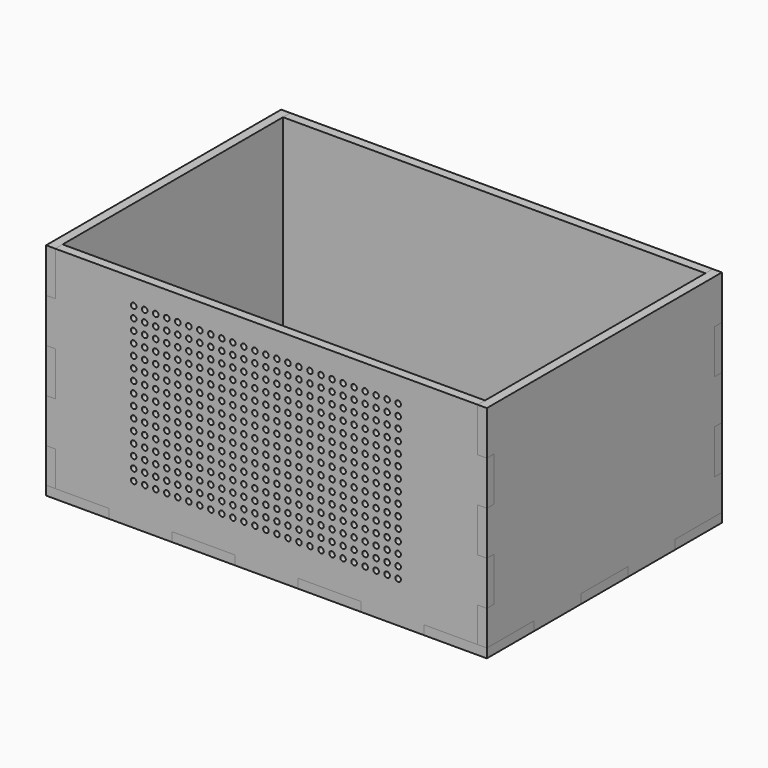
from build123d import *

# Parameters (mm, degrees)
F0_W      = 18.5964285714
F0_H      = 3.175
F0_W_2    = 3.175
F0_H_2    = 17.145
F0_H_3    = 20.32
F0_W_3    = 21.7714285714
F1_DEPTH  = 3.175
F2_W      = 3.175
F2_H      = 15.24
F2_H_2    = 12.065
F2_H_3    = 3.175
F3_DEPTH  = 3.175
F7_DEPTH  = 3.175
F10_R     = 0.9525
F11_DEPTH = 25.4


with BuildPart() as f1:
    # F0 (on Top) → F1 (new body)
    with BuildSketch(Plane.XY):
        Polygon((73.025, 30.48), (73.025, 47.625), (54.4285714286, 47.625), (32.6571428571, 47.625), (10.8857142857, 47.625), (-10.8857142857, 47.625), (-32.6571428571, 47.625), (-54.4285714286, 47.625), (-73.025, 47.625), (-73.025, 30.48), (-73.025, 10.16), (-73.025, -10.16), (-73.025, -30.48), (-73.025, -47.625), (-54.4285714286, -47.625), (-32.6571428571, -47.625), (-10.8857142857, -47.625), (10.8857142857, -47.625), (32.6571428571, -47.625), (54.4285714286, -47.625), (73.025, -47.625), (73.025, -30.48), (73.025, -10.16), (73.025, 10.16), align=None)
        with Locations((-63.7267857143, 49.2125)):
            Rectangle(F0_W, F0_H)
        with Locations((-74.6125, 49.2125)):
            Rectangle(F0_W_2, F0_H)
        with Locations((-74.6125, 39.0525)):
            Rectangle(F0_W_2, F0_H_2)
        with Locations((-74.6125, 0)):
            Rectangle(F0_W_2, F0_H_3)
        with Locations((-74.6125, -39.0525)):
            Rectangle(F0_W_2, F0_H_2)
        with Locations((-74.6125, -49.2125)):
            Rectangle(F0_W_2, F0_H)
        with Locations((-63.7267857143, -49.2125)):
            Rectangle(F0_W, F0_H)
        with Locations((-21.7714285714, -49.2125)):
            Rectangle(F0_W_3, F0_H)
        with Locations((21.7714285714, -49.2125)):
            Rectangle(F0_W_3, F0_H)
        with Locations((63.7267857143, -49.2125)):
            Rectangle(F0_W, F0_H)
        with Locations((74.6125, -49.2125)):
            Rectangle(F0_W_2, F0_H)
        with Locations((74.6125, -39.0525)):
            Rectangle(F0_W_2, F0_H_2)
        with Locations((74.6125, 0)):
            Rectangle(F0_W_2, F0_H_3)
        with Locations((74.6125, 39.0525)):
            Rectangle(F0_W_2, F0_H_2)
        with Locations((74.6125, 49.2125)):
            Rectangle(F0_W_2, F0_H)
        with Locations((63.7267857143, 49.2125)):
            Rectangle(F0_W, F0_H)
        with Locations((21.7714285714, 49.2125)):
            Rectangle(F0_W_3, F0_H)
        with Locations((-21.7714285714, 49.2125)):
            Rectangle(F0_W_3, F0_H)
    extrude(amount=F1_DEPTH)


with BuildPart() as f3:
    # F2 (on face) → F3 (new body)
    with BuildSketch(Plane.YZ.offset(76.2)):
        Polygon((-30.48, 3.175), (-30.48, 0), (47.625, 0), (47.625, 15.24), (47.625, 30.48), (47.625, 45.72), (47.625, 60.96), (47.625, 76.2), (-47.625, 76.2), (-47.625, 60.96), (-47.625, 45.72), (-47.625, 30.48), (-47.625, 15.24), (-47.625, 3.175), align=None)
        with Locations((-49.2125, 68.58)):
            Rectangle(F2_W, F2_H)
        with Locations((-49.2125, 38.1)):
            Rectangle(F2_W, F2_H)
        with Locations((-49.2125, 9.2075)):
            Rectangle(F2_W, F2_H_2)
        with Locations((49.2125, 7.62)):
            Rectangle(F2_W, F2_H)
        with Locations((49.2125, 38.1)):
            Rectangle(F2_W, F2_H)
        with Locations((49.2125, 68.58)):
            Rectangle(F2_W, F2_H)
        with Locations((-49.2125, 1.5875)):
            Rectangle(F2_W, F2_H_3)
    extrude(amount=-F3_DEPTH)

    # F4: cut F1
    add(f1.part, mode=Mode.SUBTRACT)


with BuildPart() as f5_1:
    # F5: instance of F3
    add(f3.part.mirror(Plane.YZ))


with BuildPart() as f7:
    # F6 (on face) → F7 (new body)
    with BuildSketch(Plane(origin=(0, 50.8, 0), x_dir=(-1, 0, 0), z_dir=(0, 1, 0))):
        Polygon((-54.4285714286, 3.175), (-54.4285714286, 0), (76.2, 0), (76.2, 76.2), (-76.2, 76.2), (-76.2, 3.175), align=None)
    extrude(amount=-F7_DEPTH)

    # F8: cut F5_1, F1, F3
    add(f5_1.part, mode=Mode.SUBTRACT)
    add(f1.part, mode=Mode.SUBTRACT)
    add(f3.part, mode=Mode.SUBTRACT)


with BuildPart() as f9_1:
    # F9: instance of F7
    add(f7.part.mirror(Plane.XZ))

    # F10 (on face) → F11 (cut)
    with BuildSketch(Plane.XZ.offset(50.8)):
        with Locations((-26.85742952, 18.0873329692)):
            Circle(F10_R)
        with Locations((-30.66742952, 21.8973329692)):
            Circle(F10_R)
        with Locations((-34.47742952, 25.7073329692)):
            Circle(F10_R)
        with Locations((-3.99742952, 56.1873329692)):
            Circle(F10_R)
        with Locations((-7.80742952, 59.9973329692)):
            Circle(F10_R)
        with Locations((-11.61742952, 63.8073329692)):
            Circle(F10_R)
        with Locations((-15.42742952, 67.6173329692)):
            Circle(F10_R)
        with Locations((11.24257048, 40.9473329692)):
            Circle(F10_R)
        with Locations((7.43257048, 44.7573329692)):
            Circle(F10_R)
        with Locations((3.62257048, 48.5673329692)):
            Circle(F10_R)
        with Locations((-0.18742952, 52.3773329692)):
            Circle(F10_R)
        with Locations((26.48257048, 25.7073329692)):
            Circle(F10_R)
        with Locations((22.67257048, 29.5173329692)):
            Circle(F10_R)
        with Locations((15.05257048, 37.1373329692)):
            Circle(F10_R)
        with Locations((45.53257048, 67.6173329692)):
            Circle(F10_R)
        with Locations((34.10257048, 18.0873329692)):
            Circle(F10_R)
        with Locations((30.29257048, 21.8973329692)):
            Circle(F10_R)
        with Locations((-45.90742952, 18.0873329692)):
            Circle(F10_R)
        with Locations((-45.90742952, 59.9973329692)):
            Circle(F10_R)
        with Locations((-45.90742952, 56.1873329692)):
            Circle(F10_R)
        with Locations((-45.90742952, 52.3773329692)):
            Circle(F10_R)
        with Locations((-45.90742952, 40.9473329692)):
            Circle(F10_R)
        with Locations((-45.90742952, 37.1373329692)):
            Circle(F10_R)
        with Locations((-45.90742952, 21.8973329692)):
            Circle(F10_R)
        with Locations((-30.66742952, 18.0873329692)):
            Circle(F10_R)
        with Locations((-34.47742952, 21.8973329692)):
            Circle(F10_R)
        with Locations((-3.99742952, 52.3773329692)):
            Circle(F10_R)
        with Locations((-7.80742952, 56.1873329692)):
            Circle(F10_R)
        with Locations((-11.61742952, 59.9973329692)):
            Circle(F10_R)
        with Locations((-15.42742952, 63.8073329692)):
            Circle(F10_R)
        with Locations((11.24257048, 37.1373329692)):
            Circle(F10_R)
        with Locations((7.43257048, 40.9473329692)):
            Circle(F10_R)
        with Locations((3.62257048, 44.7573329692)):
            Circle(F10_R)
        with Locations((26.48257048, 21.8973329692)):
            Circle(F10_R)
        with Locations((22.67257048, 25.7073329692)):
            Circle(F10_R)
        with Locations((45.53257048, 63.8073329692)):
            Circle(F10_R)
        with Locations((41.72257048, 67.6173329692)):
            Circle(F10_R)
        with Locations((30.29257048, 18.0873329692)):
            Circle(F10_R)
        with Locations((-7.80742952, 52.3773329692)):
            Circle(F10_R)
        with Locations((-11.61742952, 56.1873329692)):
            Circle(F10_R)
        with Locations((-15.42742952, 59.9973329692)):
            Circle(F10_R)
        with Locations((7.43257048, 37.1373329692)):
            Circle(F10_R)
        with Locations((3.62257048, 40.9473329692)):
            Circle(F10_R)
        with Locations((26.48257048, 18.0873329692)):
            Circle(F10_R)
        with Locations((22.67257048, 21.8973329692)):
            Circle(F10_R)
        with Locations((45.53257048, 59.9973329692)):
            Circle(F10_R)
        with Locations((41.72257048, 63.8073329692)):
            Circle(F10_R)
        with Locations((-38.28742952, 21.8973329692)):
            Circle(F10_R)
        with Locations((-30.66742952, 14.2773329692)):
            Circle(F10_R)
        with Locations((-34.47742952, 18.0873329692)):
            Circle(F10_R)
        with Locations((7.43257048, 33.3273329692)):
            Circle(F10_R)
        with Locations((3.62257048, 37.1373329692)):
            Circle(F10_R)
        with Locations((-0.18742952, 40.9473329692)):
            Circle(F10_R)
        with Locations((26.48257048, 14.2773329692)):
            Circle(F10_R)
        with Locations((22.67257048, 18.0873329692)):
            Circle(F10_R)
        with Locations((18.86257048, 21.8973329692)):
            Circle(F10_R)
        with Locations((45.53257048, 56.1873329692)):
            Circle(F10_R)
        with Locations((41.72257048, 59.9973329692)):
            Circle(F10_R)
        with Locations((-38.28742952, 18.0873329692)):
            Circle(F10_R)
        with Locations((-42.09742952, 21.8973329692)):
            Circle(F10_R)
        with Locations((-34.47742952, 14.2773329692)):
            Circle(F10_R)
        with Locations((-11.61742952, 52.3773329692)):
            Circle(F10_R)
        with Locations((-15.42742952, 56.1873329692)):
            Circle(F10_R)
        with Locations((22.67257048, 14.2773329692)):
            Circle(F10_R)
        with Locations((18.86257048, 18.0873329692)):
            Circle(F10_R)
        with Locations((15.05257048, 21.8973329692)):
            Circle(F10_R)
        with Locations((45.53257048, 52.3773329692)):
            Circle(F10_R)
        with Locations((41.72257048, 56.1873329692)):
            Circle(F10_R)
        with Locations((-42.09742952, 18.0873329692)):
            Circle(F10_R)
        with Locations((-19.23742952, 56.1873329692)):
            Circle(F10_R)
        with Locations((-30.66742952, 67.6173329692)):
            Circle(F10_R)
        with Locations((-3.99742952, 40.9473329692)):
            Circle(F10_R)
        with Locations((-11.61742952, 48.5673329692)):
            Circle(F10_R)
        with Locations((-15.42742952, 52.3773329692)):
            Circle(F10_R)
        with Locations((7.43257048, 29.5173329692)):
            Circle(F10_R)
        with Locations((3.62257048, 33.3273329692)):
            Circle(F10_R)
        with Locations((-0.18742952, 37.1373329692)):
            Circle(F10_R)
        with Locations((-30.66742952, 44.7573329692)):
            Circle(F10_R)
        with Locations((-34.47742952, 48.5673329692)):
            Circle(F10_R)
        with Locations((-38.28742952, 52.3773329692)):
            Circle(F10_R)
        with Locations((-42.09742952, 56.1873329692)):
            Circle(F10_R)
        with Locations((-15.42742952, 29.5173329692)):
            Circle(F10_R)
        with Locations((-23.04742952, 37.1373329692)):
            Circle(F10_R)
        with Locations((-26.85742952, 40.9473329692)):
            Circle(F10_R)
        with Locations((-3.99742952, 18.0873329692)):
            Circle(F10_R)
        with Locations((-7.80742952, 21.8973329692)):
            Circle(F10_R)
        with Locations((-11.61742952, 25.7073329692)):
            Circle(F10_R)
        with Locations((18.86257048, 56.1873329692)):
            Circle(F10_R)
        with Locations((7.43257048, 67.6173329692)):
            Circle(F10_R)
        with Locations((34.10257048, 40.9473329692)):
            Circle(F10_R)
        with Locations((26.48257048, 48.5673329692)):
            Circle(F10_R)
        with Locations((22.67257048, 52.3773329692)):
            Circle(F10_R)
        with Locations((45.53257048, 29.5173329692)):
            Circle(F10_R)
        with Locations((41.72257048, 33.3273329692)):
            Circle(F10_R)
        with Locations((37.91257048, 37.1373329692)):
            Circle(F10_R)
        with Locations((-30.66742952, 40.9473329692)):
            Circle(F10_R)
        with Locations((-34.47742952, 44.7573329692)):
            Circle(F10_R)
        with Locations((-42.09742952, 52.3773329692)):
            Circle(F10_R)
        with Locations((-26.85742952, 52.3773329692)):
            Circle(F10_R)
        with Locations((-30.66742952, 56.1873329692)):
            Circle(F10_R)
        with Locations((-34.47742952, 59.9973329692)):
            Circle(F10_R)
        with Locations((-11.61742952, 37.1373329692)):
            Circle(F10_R)
        with Locations((-15.42742952, 40.9473329692)):
            Circle(F10_R)
        with Locations((3.62257048, 21.8973329692)):
            Circle(F10_R)
        with Locations((22.67257048, 63.8073329692)):
            Circle(F10_R)
        with Locations((7.43257048, 18.0873329692)):
            Circle(F10_R)
        with Locations((34.10257048, 52.3773329692)):
            Circle(F10_R)
        with Locations((30.29257048, 56.1873329692)):
            Circle(F10_R)
        with Locations((26.48257048, 59.9973329692)):
            Circle(F10_R)
        with Locations((45.53257048, 40.9473329692)):
            Circle(F10_R)
        with Locations((41.72257048, 44.7573329692)):
            Circle(F10_R)
        with Locations((-15.42742952, 25.7073329692)):
            Circle(F10_R)
        with Locations((-26.85742952, 37.1373329692)):
            Circle(F10_R)
        with Locations((3.62257048, 67.6173329692)):
            Circle(F10_R)
        with Locations((-30.66742952, 63.8073329692)):
            Circle(F10_R)
        with Locations((-7.80742952, 18.0873329692)):
            Circle(F10_R)
        with Locations((-34.47742952, 67.6173329692)):
            Circle(F10_R)
        with Locations((-11.61742952, 21.8973329692)):
            Circle(F10_R)
        with Locations((-15.42742952, 48.5673329692)):
            Circle(F10_R)
        with Locations((-19.23742952, 52.3773329692)):
            Circle(F10_R)
        with Locations((-23.04742952, 56.1873329692)):
            Circle(F10_R)
        with Locations((-26.85742952, 59.9973329692)):
            Circle(F10_R)
        with Locations((18.86257048, 52.3773329692)):
            Circle(F10_R)
        with Locations((15.05257048, 56.1873329692)):
            Circle(F10_R)
        with Locations((11.24257048, 59.9973329692)):
            Circle(F10_R)
        with Locations((-3.99742952, 37.1373329692)):
            Circle(F10_R)
        with Locations((-7.80742952, 40.9473329692)):
            Circle(F10_R)
        with Locations((-11.61742952, 44.7573329692)):
            Circle(F10_R)
        with Locations((15.05257048, 18.0873329692)):
            Circle(F10_R)
        with Locations((11.24257048, 21.8973329692)):
            Circle(F10_R)
        with Locations((7.43257048, 25.7073329692)):
            Circle(F10_R)
        with Locations((3.62257048, 29.5173329692)):
            Circle(F10_R)
        with Locations((26.48257048, 67.6173329692)):
            Circle(F10_R)
        with Locations((45.53257048, 48.5673329692)):
            Circle(F10_R)
        with Locations((41.72257048, 52.3773329692)):
            Circle(F10_R)
        with Locations((7.43257048, 63.8073329692)):
            Circle(F10_R)
        with Locations((34.10257048, 37.1373329692)):
            Circle(F10_R)
        with Locations((30.29257048, 40.9473329692)):
            Circle(F10_R)
        with Locations((37.91257048, 56.1873329692)):
            Circle(F10_R)
        with Locations((26.48257048, 44.7573329692)):
            Circle(F10_R)
        with Locations((22.67257048, 48.5673329692)):
            Circle(F10_R)
        with Locations((45.53257048, 25.7073329692)):
            Circle(F10_R)
        with Locations((41.72257048, 29.5173329692)):
            Circle(F10_R)
        with Locations((-30.66742952, 59.9973329692)):
            Circle(F10_R)
        with Locations((-34.47742952, 63.8073329692)):
            Circle(F10_R)
        with Locations((-30.66742952, 37.1373329692)):
            Circle(F10_R)
        with Locations((-15.42742952, 44.7573329692)):
            Circle(F10_R)
        with Locations((-23.04742952, 52.3773329692)):
            Circle(F10_R)
        with Locations((-26.85742952, 56.1873329692)):
            Circle(F10_R)
        with Locations((-7.80742952, 37.1373329692)):
            Circle(F10_R)
        with Locations((-11.61742952, 40.9473329692)):
            Circle(F10_R)
        with Locations((-34.47742952, 40.9473329692)):
            Circle(F10_R)
        with Locations((-15.42742952, 21.8973329692)):
            Circle(F10_R)
        with Locations((11.24257048, 18.0873329692)):
            Circle(F10_R)
        with Locations((7.43257048, 21.8973329692)):
            Circle(F10_R)
        with Locations((3.62257048, 25.7073329692)):
            Circle(F10_R)
        with Locations((34.10257048, 56.1873329692)):
            Circle(F10_R)
        with Locations((30.29257048, 59.9973329692)):
            Circle(F10_R)
        with Locations((26.48257048, 63.8073329692)):
            Circle(F10_R)
        with Locations((22.67257048, 67.6173329692)):
            Circle(F10_R)
        with Locations((45.53257048, 44.7573329692)):
            Circle(F10_R)
        with Locations((41.72257048, 48.5673329692)):
            Circle(F10_R)
        with Locations((37.91257048, 52.3773329692)):
            Circle(F10_R)
        with Locations((-30.66742952, 52.3773329692)):
            Circle(F10_R)
        with Locations((-34.47742952, 56.1873329692)):
            Circle(F10_R)
        with Locations((-15.42742952, 37.1373329692)):
            Circle(F10_R)
        with Locations((-19.23742952, 40.9473329692)):
            Circle(F10_R)
        with Locations((-0.18742952, 21.8973329692)):
            Circle(F10_R)
        with Locations((-11.61742952, 33.3273329692)):
            Circle(F10_R)
        with Locations((7.43257048, 14.2773329692)):
            Circle(F10_R)
        with Locations((3.62257048, 18.0873329692)):
            Circle(F10_R)
        with Locations((30.29257048, 52.3773329692)):
            Circle(F10_R)
        with Locations((26.48257048, 56.1873329692)):
            Circle(F10_R)
        with Locations((22.67257048, 59.9973329692)):
            Circle(F10_R)
        with Locations((41.72257048, 40.9473329692)):
            Circle(F10_R)
        with Locations((45.53257048, 37.1373329692)):
            Circle(F10_R)
        with Locations((3.62257048, 63.8073329692)):
            Circle(F10_R)
        with Locations((-30.66742952, 48.5673329692)):
            Circle(F10_R)
        with Locations((-34.47742952, 52.3773329692)):
            Circle(F10_R)
        with Locations((-38.28742952, 56.1873329692)):
            Circle(F10_R)
        with Locations((-11.61742952, 18.0873329692)):
            Circle(F10_R)
        with Locations((15.05257048, 52.3773329692)):
            Circle(F10_R)
        with Locations((11.24257048, 56.1873329692)):
            Circle(F10_R)
        with Locations((7.43257048, 59.9973329692)):
            Circle(F10_R)
        with Locations((30.29257048, 37.1373329692)):
            Circle(F10_R)
        with Locations((26.48257048, 40.9473329692)):
            Circle(F10_R)
        with Locations((22.67257048, 44.7573329692)):
            Circle(F10_R)
        with Locations((45.53257048, 21.8973329692)):
            Circle(F10_R)
        with Locations((41.72257048, 25.7073329692)):
            Circle(F10_R)
        with Locations((-15.42742952, 33.3273329692)):
            Circle(F10_R)
        with Locations((-19.23742952, 37.1373329692)):
            Circle(F10_R)
        with Locations((-23.04742952, 40.9473329692)):
            Circle(F10_R)
        with Locations((-0.18742952, 18.0873329692)):
            Circle(F10_R)
        with Locations((-3.99742952, 21.8973329692)):
            Circle(F10_R)
        with Locations((-11.61742952, 29.5173329692)):
            Circle(F10_R)
        with Locations((3.62257048, 14.2773329692)):
            Circle(F10_R)
        with Locations((26.48257048, 52.3773329692)):
            Circle(F10_R)
        with Locations((22.67257048, 56.1873329692)):
            Circle(F10_R)
        with Locations((45.53257048, 33.3273329692)):
            Circle(F10_R)
        with Locations((41.72257048, 37.1373329692)):
            Circle(F10_R)
        with Locations((37.91257048, 40.9473329692)):
            Circle(F10_R)
        with Locations((-30.66742952, 33.3273329692)):
            Circle(F10_R)
        with Locations((-34.47742952, 37.1373329692)):
            Circle(F10_R)
        with Locations((-38.28742952, 40.9473329692)):
            Circle(F10_R)
        with Locations((-15.42742952, 18.0873329692)):
            Circle(F10_R)
        with Locations((-19.23742952, 21.8973329692)):
            Circle(F10_R)
        with Locations((3.62257048, 59.9973329692)):
            Circle(F10_R)
        with Locations((-11.61742952, 14.2773329692)):
            Circle(F10_R)
        with Locations((11.24257048, 52.3773329692)):
            Circle(F10_R)
        with Locations((7.43257048, 56.1873329692)):
            Circle(F10_R)
        with Locations((26.48257048, 37.1373329692)):
            Circle(F10_R)
        with Locations((22.67257048, 40.9473329692)):
            Circle(F10_R)
        with Locations((45.53257048, 18.0873329692)):
            Circle(F10_R)
        with Locations((41.72257048, 21.8973329692)):
            Circle(F10_R)
        with Locations((-38.28742952, 37.1373329692)):
            Circle(F10_R)
        with Locations((-42.09742952, 40.9473329692)):
            Circle(F10_R)
        with Locations((-23.04742952, 21.8973329692)):
            Circle(F10_R)
        with Locations((-30.66742952, 29.5173329692)):
            Circle(F10_R)
        with Locations((-34.47742952, 33.3273329692)):
            Circle(F10_R)
        with Locations((-15.42742952, 14.2773329692)):
            Circle(F10_R)
        with Locations((-19.23742952, 18.0873329692)):
            Circle(F10_R)
        with Locations((7.43257048, 52.3773329692)):
            Circle(F10_R)
        with Locations((3.62257048, 56.1873329692)):
            Circle(F10_R)
        with Locations((26.48257048, 33.3273329692)):
            Circle(F10_R)
        with Locations((22.67257048, 37.1373329692)):
            Circle(F10_R)
        with Locations((18.86257048, 40.9473329692)):
            Circle(F10_R)
        with Locations((41.72257048, 18.0873329692)):
            Circle(F10_R)
        with Locations((37.91257048, 21.8973329692)):
            Circle(F10_R)
        with Locations((45.53257048, 14.2773329692)):
            Circle(F10_R)
        with Locations((-23.04742952, 18.0873329692)):
            Circle(F10_R)
        with Locations((-42.09742952, 37.1373329692)):
            Circle(F10_R)
        with Locations((-26.85742952, 21.8973329692)):
            Circle(F10_R)
        with Locations((-30.66742952, 25.7073329692)):
            Circle(F10_R)
        with Locations((-34.47742952, 29.5173329692)):
            Circle(F10_R)
        with Locations((-11.61742952, 67.6173329692)):
            Circle(F10_R)
        with Locations((7.43257048, 48.5673329692)):
            Circle(F10_R)
        with Locations((3.62257048, 52.3773329692)):
            Circle(F10_R)
        with Locations((26.48257048, 29.5173329692)):
            Circle(F10_R)
        with Locations((-0.18742952, 56.1873329692)):
            Circle(F10_R)
        with Locations((22.67257048, 33.3273329692)):
            Circle(F10_R)
        with Locations((18.86257048, 37.1373329692)):
            Circle(F10_R)
        with Locations((15.05257048, 40.9473329692)):
            Circle(F10_R)
        with Locations((41.72257048, 14.2773329692)):
            Circle(F10_R)
        with Locations((37.91257048, 18.0873329692)):
            Circle(F10_R)
        with Locations((34.10257048, 21.8973329692)):
            Circle(F10_R)
        with Locations((-38.28742952, 29.5173329692)):
            Circle(F10_R)
        with Locations((-42.09742952, 33.3273329692)):
            Circle(F10_R)
        with Locations((-23.04742952, 14.2773329692)):
            Circle(F10_R)
        with Locations((18.86257048, 33.3273329692)):
            Circle(F10_R)
        with Locations((37.91257048, 14.2773329692)):
            Circle(F10_R)
        with Locations((-42.09742952, 67.6173329692)):
            Circle(F10_R)
        with Locations((-45.90742952, 14.2773329692)):
            Circle(F10_R)
        with Locations((-45.90742952, 67.6173329692)):
            Circle(F10_R)
        with Locations((-45.90742952, 63.8073329692)):
            Circle(F10_R)
        with Locations((-45.90742952, 48.5673329692)):
            Circle(F10_R)
        with Locations((-45.90742952, 44.7573329692)):
            Circle(F10_R)
        with Locations((-45.90742952, 33.3273329692)):
            Circle(F10_R)
        with Locations((-45.90742952, 29.5173329692)):
            Circle(F10_R)
        with Locations((-45.90742952, 25.7073329692)):
            Circle(F10_R)
        with Locations((-19.23742952, 67.6173329692)):
            Circle(F10_R)
        with Locations((-26.85742952, 14.2773329692)):
            Circle(F10_R)
        with Locations((-0.18742952, 48.5673329692)):
            Circle(F10_R)
        with Locations((18.86257048, 29.5173329692)):
            Circle(F10_R)
        with Locations((15.05257048, 33.3273329692)):
            Circle(F10_R)
        with Locations((34.10257048, 14.2773329692)):
            Circle(F10_R)
        with Locations((-42.09742952, 29.5173329692)):
            Circle(F10_R)
        with Locations((-38.28742952, 25.7073329692)):
            Circle(F10_R)
        with Locations((-3.99742952, 48.5673329692)):
            Circle(F10_R)
        with Locations((11.24257048, 33.3273329692)):
            Circle(F10_R)
        with Locations((-0.18742952, 44.7573329692)):
            Circle(F10_R)
        with Locations((18.86257048, 25.7073329692)):
            Circle(F10_R)
        with Locations((15.05257048, 29.5173329692)):
            Circle(F10_R)
        with Locations((37.91257048, 67.6173329692)):
            Circle(F10_R)
        with Locations((30.29257048, 14.2773329692)):
            Circle(F10_R)
        with Locations((-42.09742952, 25.7073329692)):
            Circle(F10_R)
        with Locations((-19.23742952, 63.8073329692)):
            Circle(F10_R)
        with Locations((-23.04742952, 67.6173329692)):
            Circle(F10_R)
        with Locations((11.24257048, 29.5173329692)):
            Circle(F10_R)
        with Locations((15.05257048, 25.7073329692)):
            Circle(F10_R)
        with Locations((37.91257048, 63.8073329692)):
            Circle(F10_R)
        with Locations((34.10257048, 67.6173329692)):
            Circle(F10_R)
        with Locations((-19.23742952, 59.9973329692)):
            Circle(F10_R)
        with Locations((-23.04742952, 63.8073329692)):
            Circle(F10_R)
        with Locations((-26.85742952, 67.6173329692)):
            Circle(F10_R)
        with Locations((-3.99742952, 44.7573329692)):
            Circle(F10_R)
        with Locations((-7.80742952, 48.5673329692)):
            Circle(F10_R)
        with Locations((30.29257048, 67.6173329692)):
            Circle(F10_R)
        with Locations((37.91257048, 59.9973329692)):
            Circle(F10_R)
        with Locations((34.10257048, 63.8073329692)):
            Circle(F10_R)
        with Locations((-38.28742952, 14.2773329692)):
            Circle(F10_R)
        with Locations((-23.04742952, 59.9973329692)):
            Circle(F10_R)
        with Locations((-26.85742952, 63.8073329692)):
            Circle(F10_R)
        with Locations((-7.80742952, 44.7573329692)):
            Circle(F10_R)
        with Locations((11.24257048, 25.7073329692)):
            Circle(F10_R)
        with Locations((-19.23742952, 33.3273329692)):
            Circle(F10_R)
        with Locations((-0.18742952, 14.2773329692)):
            Circle(F10_R)
        with Locations((15.05257048, 59.9973329692)):
            Circle(F10_R)
        with Locations((11.24257048, 63.8073329692)):
            Circle(F10_R)
        with Locations((30.29257048, 44.7573329692)):
            Circle(F10_R)
        with Locations((-38.28742952, 48.5673329692)):
            Circle(F10_R)
        with Locations((-38.28742952, 63.8073329692)):
            Circle(F10_R)
        with Locations((-19.23742952, 44.7573329692)):
            Circle(F10_R)
        with Locations((-23.04742952, 48.5673329692)):
            Circle(F10_R)
        with Locations((-0.18742952, 25.7073329692)):
            Circle(F10_R)
        with Locations((-3.99742952, 29.5173329692)):
            Circle(F10_R)
        with Locations((-7.80742952, 33.3273329692)):
            Circle(F10_R)
        with Locations((18.86257048, 67.6173329692)):
            Circle(F10_R)
        with Locations((11.24257048, 14.2773329692)):
            Circle(F10_R)
        with Locations((37.91257048, 48.5673329692)):
            Circle(F10_R)
        with Locations((-19.23742952, 29.5173329692)):
            Circle(F10_R)
        with Locations((-23.04742952, 33.3273329692)):
            Circle(F10_R)
        with Locations((-3.99742952, 14.2773329692)):
            Circle(F10_R)
        with Locations((-42.09742952, 14.2773329692)):
            Circle(F10_R)
        with Locations((-0.18742952, 33.3273329692)):
            Circle(F10_R)
        with Locations((34.10257048, 59.9973329692)):
            Circle(F10_R)
        with Locations((30.29257048, 63.8073329692)):
            Circle(F10_R)
        with Locations((18.86257048, 14.2773329692)):
            Circle(F10_R)
        with Locations((37.91257048, 33.3273329692)):
            Circle(F10_R)
        with Locations((-38.28742952, 67.6173329692)):
            Circle(F10_R)
        with Locations((-19.23742952, 48.5673329692)):
            Circle(F10_R)
        with Locations((-0.18742952, 29.5173329692)):
            Circle(F10_R)
        with Locations((-3.99742952, 33.3273329692)):
            Circle(F10_R)
        with Locations((-38.28742952, 44.7573329692)):
            Circle(F10_R)
        with Locations((-42.09742952, 48.5673329692)):
            Circle(F10_R)
        with Locations((-19.23742952, 25.7073329692)):
            Circle(F10_R)
        with Locations((15.05257048, 14.2773329692)):
            Circle(F10_R)
        with Locations((-23.04742952, 29.5173329692)):
            Circle(F10_R)
        with Locations((-26.85742952, 33.3273329692)):
            Circle(F10_R)
        with Locations((-38.28742952, 59.9973329692)):
            Circle(F10_R)
        with Locations((-42.09742952, 63.8073329692)):
            Circle(F10_R)
        with Locations((-23.04742952, 44.7573329692)):
            Circle(F10_R)
        with Locations((-26.85742952, 48.5673329692)):
            Circle(F10_R)
        with Locations((-3.99742952, 25.7073329692)):
            Circle(F10_R)
        with Locations((-7.80742952, 29.5173329692)):
            Circle(F10_R)
        with Locations((18.86257048, 63.8073329692)):
            Circle(F10_R)
        with Locations((15.05257048, 67.6173329692)):
            Circle(F10_R)
        with Locations((34.10257048, 48.5673329692)):
            Circle(F10_R)
        with Locations((37.91257048, 44.7573329692)):
            Circle(F10_R)
        with Locations((-0.18742952, 67.6173329692)):
            Circle(F10_R)
        with Locations((-7.80742952, 14.2773329692)):
            Circle(F10_R)
        with Locations((-42.09742952, 59.9973329692)):
            Circle(F10_R)
        with Locations((18.86257048, 48.5673329692)):
            Circle(F10_R)
        with Locations((34.10257048, 33.3273329692)):
            Circle(F10_R)
        with Locations((37.91257048, 29.5173329692)):
            Circle(F10_R)
        with Locations((-26.85742952, 44.7573329692)):
            Circle(F10_R)
        with Locations((-7.80742952, 25.7073329692)):
            Circle(F10_R)
        with Locations((18.86257048, 59.9973329692)):
            Circle(F10_R)
        with Locations((15.05257048, 63.8073329692)):
            Circle(F10_R)
        with Locations((11.24257048, 67.6173329692)):
            Circle(F10_R)
        with Locations((34.10257048, 44.7573329692)):
            Circle(F10_R)
        with Locations((30.29257048, 48.5673329692)):
            Circle(F10_R)
        with Locations((-42.09742952, 44.7573329692)):
            Circle(F10_R)
        with Locations((-23.04742952, 25.7073329692)):
            Circle(F10_R)
        with Locations((-26.85742952, 29.5173329692)):
            Circle(F10_R)
        with Locations((-0.18742952, 63.8073329692)):
            Circle(F10_R)
        with Locations((-3.99742952, 67.6173329692)):
            Circle(F10_R)
        with Locations((18.86257048, 44.7573329692)):
            Circle(F10_R)
        with Locations((15.05257048, 48.5673329692)):
            Circle(F10_R)
        with Locations((34.10257048, 29.5173329692)):
            Circle(F10_R)
        with Locations((30.29257048, 33.3273329692)):
            Circle(F10_R)
        with Locations((37.91257048, 25.7073329692)):
            Circle(F10_R)
        with Locations((-26.85742952, 25.7073329692)):
            Circle(F10_R)
        with Locations((-3.99742952, 63.8073329692)):
            Circle(F10_R)
        with Locations((-7.80742952, 67.6173329692)):
            Circle(F10_R)
        with Locations((11.24257048, 48.5673329692)):
            Circle(F10_R)
        with Locations((-0.18742952, 59.9973329692)):
            Circle(F10_R)
        with Locations((15.05257048, 44.7573329692)):
            Circle(F10_R)
        with Locations((34.10257048, 25.7073329692)):
            Circle(F10_R)
        with Locations((30.29257048, 29.5173329692)):
            Circle(F10_R)
        with Locations((-38.28742952, 33.3273329692)):
            Circle(F10_R)
        with Locations((-3.99742952, 59.9973329692)):
            Circle(F10_R)
        with Locations((-7.80742952, 63.8073329692)):
            Circle(F10_R)
        with Locations((-19.23742952, 14.2773329692)):
            Circle(F10_R)
        with Locations((11.24257048, 44.7573329692)):
            Circle(F10_R)
        with Locations((30.29257048, 25.7073329692)):
            Circle(F10_R)
    extrude(amount=-F11_DEPTH, mode=Mode.SUBTRACT)


solid = Compound([f1.part, f3.part, f5_1.part, f7.part, f9_1.part])
